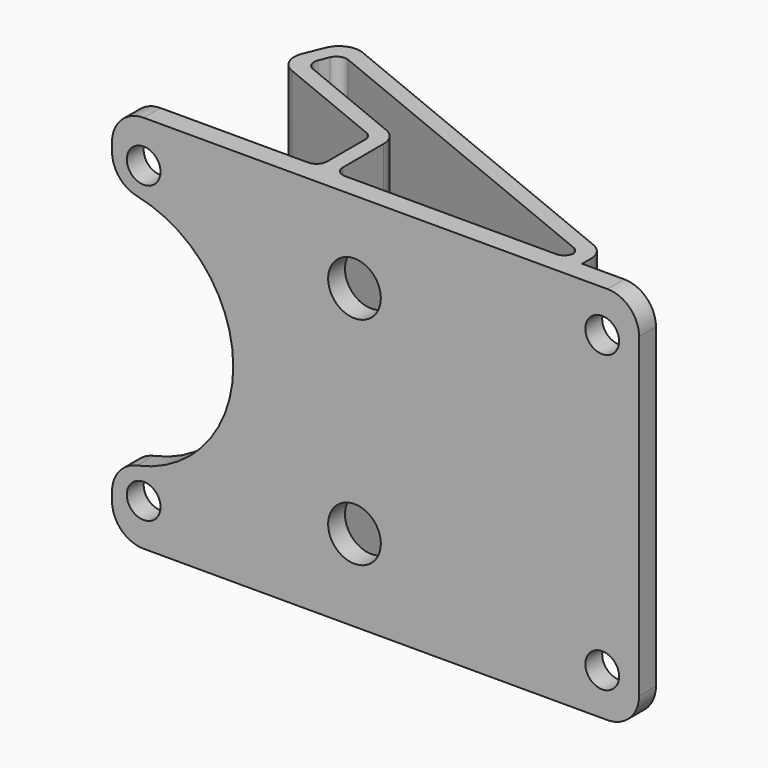
from build123d import *

# Parameters (mm, degrees)
F1_DEPTH     = 36
F2_T         = -1.5
F3_R         = 1.6
F4_DEPTH     = 1.5
F5_R         = 1.6
F6_DEPTH     = 5
F7_DEPTH     = 0.5
F8_DEPTH     = 0.5
F9_R         = 3
F10_T1_DEPTH = 36
F11_R        = 2
F5_R_2       = 2.5
F12_DEPTH    = 5


# Not quite as in the source:
# - a fillet or chamfer that OpenCascade refuses, or shapes differently, is made with other operations: its cross-section is extruded or revolved along the edge and cut away or added


with BuildPart() as f1:
    # F0 (on Top) → F1 (new body)
    with BuildSketch(Plane.XY):
        Polygon((-12, 0), (20, 0), (20, 1.5), (13, 1.5), (13, 4.3777777778), (-22.720401141, 19.0628315802), (-25, 13.5178613825), (-12, 8.1734169381), (-12, 1.5), (-30, 1.5), (-30, 0), align=None)
    extrude(amount=F1_DEPTH)

    # F2: a shell. OpenCascade refuses it in one call, so the cavity is built on its own and cut out:
    # the body offset inwards by the wall thickness, plus a prism from it out through each open face.
    f2_core = offset(f1.part, amount=F2_T, kind=Kind.INTERSECTION, mode=Mode.PRIVATE)
    f2_exits = [f2_core.faces().sort_by_distance(p)[0] for p in [
        (-5.203768, 6.959906, 34.5),
        (-5.203768, 6.959906, 1.5),
    ]]
    add(f2_core, mode=Mode.SUBTRACT)
    extrude(f2_exits, amount=-F2_T, mode=Mode.SUBTRACT)

    # F3 (on face) → F4 (cut)
    with BuildSketch(Plane(origin=(0, 1.5, 0), x_dir=(-1, 0, 0), z_dir=(0, 1, 0))):
        with Locations((-16.5, 32)):
            Circle(F3_R)
        with Locations((-16.5, 4)):
            Circle(F3_R)
    extrude(amount=-F4_DEPTH, mode=Mode.SUBTRACT)

    # F5 (on face) → F6 (cut)
    with BuildSketch(Plane.XZ):
        with Locations((-27, 32)):
            Circle(F5_R)
        with BuildLine():
            Line((-30, 29.5), (-30, 6.5))
            ThreePointArc((-30, 6.5), (-18.5, 18), (-30, 29.5))
        make_face()
        with Locations((-27, 4)):
            Circle(F5_R)
    extrude(amount=-F6_DEPTH, mode=Mode.SUBTRACT)

    # F7 (add): faces of the model
    f7_faces = [f1.faces().sort_by_distance(p)[0] for p in [
        (16.5, 1.5, 18),
        (-21, 1.5, 0.4024922359),
    ]]
    extrude(f7_faces, amount=F7_DEPTH)

    # F8 (add): a face of the model
    f8_faces = [f1.faces().sort_by_distance(p)[0] for p in [
        (0.5, 1.5, 18),
    ]]
    extrude(f8_faces, amount=F8_DEPTH)

    # F9
    f9_edges = [f1.edges().sort_by_distance(p)[0] for p in [
        (20, 1, 36),
        (20, 1, 0),
        (-30, 1, 0),
        (-30, 1, 36),
        (-30, 1, 6.5),
        (-30, 1, 29.5),
    ]]
    fillet(f9_edges, radius=F9_R)

    # F10: fillet of radius 1 on 8 edges, made by hand

    # F10_s2 → F10_t1 (join)
    with BuildSketch(Plane.XY):
        with BuildLine():
            ThreePointArc((-10.5, 3), (-10.2071067812, 2.2928932188), (-9.5, 2))
            Line((-9.5, 2), (-10.5, 2))
            Line((-10.5, 2), (-10.5, 3))
        make_face()
        with BuildLine():
            ThreePointArc((-22.1174237286, 13.954615363), (-22.6600526413, 14.4943748472), (-22.6620816337, 15.2597390224))
            Line((-22.6620816337, 15.2597390224), (-23.0423145109, 14.3348482402))
            Line((-23.0423145109, 14.3348482402), (-22.1174237286, 13.954615363))
        make_face()
        with BuildLine():
            ThreePointArc((-22.2836471604, 16.1802553088), (-21.7438876763, 16.7228842215), (-20.978523501, 16.7249132139))
            Line((-20.978523501, 16.7249132139), (-21.9034142833, 17.105146091))
            Line((-21.9034142833, 17.105146091), (-22.2836471604, 16.1802553088))
        make_face()
        with BuildLine():
            ThreePointArc((10.8802328772, 3.6274244806), (11.3307324711, 3.2592055599), (11.5, 2.7025336984))
            Line((11.5, 2.7025336984), (11.5, 3.3726313301))
            Line((11.5, 3.3726313301), (10.8802328772, 3.6274244806))
        make_face()
        with BuildLine():
            ThreePointArc((-13, 2), (-12.2928932188, 2.2928932188), (-12, 3))
            Line((-12, 3), (-12, 2))
            Line((-12, 2), (-13, 2))
        make_face()
        with BuildLine():
            ThreePointArc((-12, 7.5033193063), (-12.1692675289, 8.0599911678), (-12.6197671228, 8.4282100886))
            Line((-12.6197671228, 8.4282100886), (-12, 8.1734169381))
            Line((-12, 8.1734169381), (-12, 7.5033193063))
        make_face()
        with BuildLine():
            ThreePointArc((11.5, 3), (11.2071067812, 2.2928932188), (10.5, 2))
            Line((10.5, 2), (11.5, 2))
            Line((11.5, 2), (11.5, 3))
        make_face()
    extrude(amount=F10_T1_DEPTH)

    # F11
    f11_edges = [f1.edges().sort_by_distance(p)[0] for p in [
        (-25, 13.517861, 18),
        (-22.720401, 19.062832, 18),
        (13, 4.377778, 18),
        (-10.5, 9.178563, 18),
    ]]
    fillet(f11_edges, radius=F11_R)

    # F5 (on face) → F12 (cut)
    with BuildSketch(Plane.XZ):
        with Locations((-7, 28.25)):
            Circle(F5_R_2)
        with Locations((-7, 7.75)):
            Circle(F5_R_2)
    extrude(amount=-F12_DEPTH, mode=Mode.SUBTRACT)


solid = f1.part
